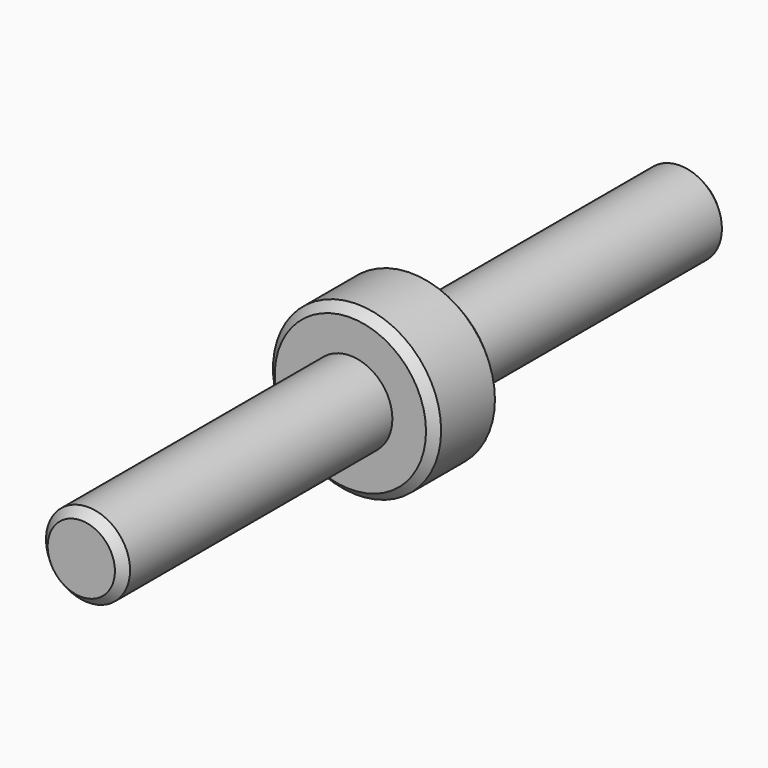
from build123d import *

# Parameters (mm, degrees)
F0_R     = 3.175
F1_DEPTH = 28.575
F0_R_2   = 6.35
F2_DEPTH = 3.175
F3_SIZE  = 0.635


with BuildPart() as f1:
    # F0 (on Front) → F1 (new body, symmetric)
    with BuildSketch(Plane.XZ):
        Circle(F0_R)
    extrude(amount=F1_DEPTH, both=True)

    # F0 (on Front) → F2 (join, symmetric)
    with BuildSketch(Plane.XZ):
        Circle(F0_R_2)
        Circle(F0_R, mode=Mode.SUBTRACT)
    extrude(amount=F2_DEPTH, both=True)

    # F3
    f3_edges = [f1.edges().sort_by_distance(p)[0] for p in [
        (-3.175, -28.575, 0),
        (-3.175, 28.575, 0),
        (-6.35, -3.175, 0),
        (-6.35, 3.175, 0),
    ]]
    chamfer(f3_edges, length=F3_SIZE)


solid = f1.part
